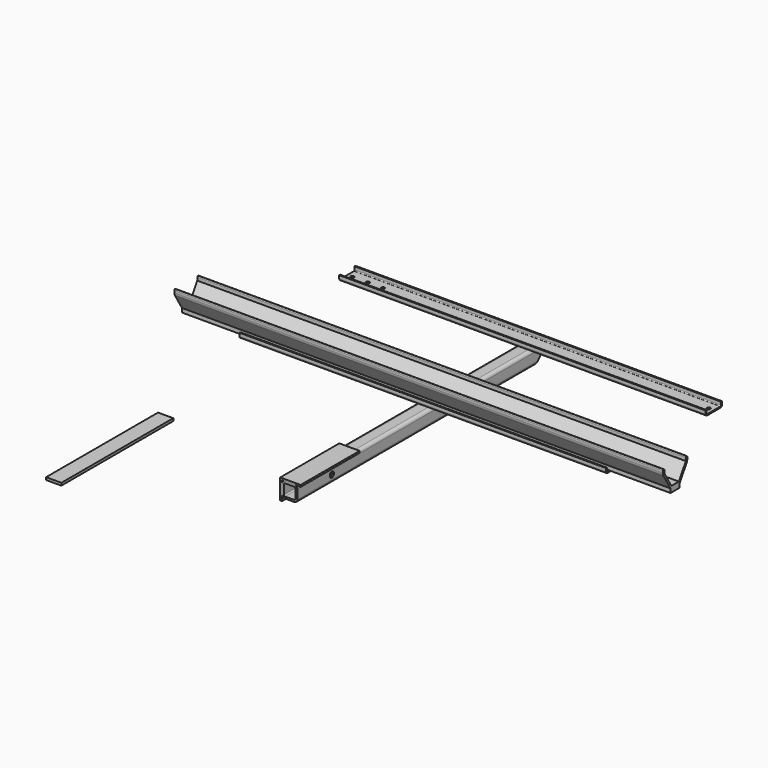
from build123d import *

# Parameters (mm, degrees)
F0_W         = 38.1
F0_H         = 38.1
F1_DEPTH     = 781.05
F2_R         = 7.62
F3_T         = -4.6228
F5_DEPTH     = 19.05
F7_DEPTH     = 184.15
F9_D         = 13.49248
F9_2_D       = 13.49248
F10_W        = 50.8
F10_H        = 12.7
F11_DEPTH    = 457.2
F12_R        = 5.08
F13_T        = -2.9972
F15_D        = 8.4328
F17_ANGLE    = 180
F18_W        = 38.1
F18_H        = 349.25
F19_DEPTH    = 6.35
F21_DEPTH    = 609.6
F22_T        = -4.572
F20_W        = 28.575
F20_H        = 10.1452730596
F23_DEPTH    = 609.6
F24_T1_DEPTH = 1231.9
F25_R        = 12.7
F27_DEPTH    = 7.62


# Not quite as in the source:
# - a fillet or chamfer that OpenCascade refuses, or shapes differently, is made with other operations: its cross-section is extruded or revolved along the edge and cut away or added


with BuildPart() as f1:
    # F0 (on Front) → F1 (new body)
    with BuildSketch(Plane.XZ):
        Rectangle(F0_W, F0_H)
    extrude(amount=-F1_DEPTH)

    # F2
    f2_edges = [f1.edges().sort_by_distance(p)[0] for p in [
        (-19.05, 390.525, -19.05),
        (-19.05, 390.525, 19.05),
        (19.05, 390.525, -19.05),
        (19.05, 390.525, 19.05),
    ]]
    fillet(f2_edges, radius=F2_R)

    # F3
    f3_openings = [f1.faces().sort_by_distance(p)[0] for p in [
        (0, 781.05, 0),
        (0, 0, 0),
    ]]
    offset(amount=F3_T, openings=f3_openings)

    # F4 (on Right) → F5 (cut, symmetric)
    with BuildSketch(Plane.YZ):
        Polygon((781.05, -19.05), (781.05, -14.4272), (781.05, 14.4272), (781.05, 19.05), (742.95, -19.05), align=None)
    extrude(amount=F5_DEPTH, both=True, mode=Mode.SUBTRACT)

    # F9 (through all)
    with Locations(Plane.YZ.offset(19.05)):
        with Locations((107.95, 0)):
            Hole(F9_D / 2)


with BuildPart() as f7:
    # F6 (on Front) → F7 (new body)
    with BuildSketch(Plane.XZ):
        Polygon((27.178, 23.622), (-23.622, 23.622), (-23.622, -27.178), (-19.05, -27.178), (-19.05, 19.05), (27.178, 19.05), align=None)
    extrude(amount=-F7_DEPTH)

    # F9#2 (through all)
    with Locations(Plane.YZ.offset(19.05)):
        with Locations((107.95, 0)):
            Hole(F9_2_D / 2)


with BuildPart() as f11:
    # F10 (on Right) → F11 (new body, symmetric)
    with BuildSketch(Plane.YZ):
        with Locations((751.332, 25.4)):
            Rectangle(F10_W, F10_H)
    extrude(amount=F11_DEPTH, both=True)

    # F12
    f12_edges = [f11.edges().sort_by_distance(p)[0] for p in [
        (0, 725.932, 19.05),
        (0, 776.732, 19.05),
    ]]
    fillet(f12_edges, radius=F12_R)

    # F13
    f13_openings = [f11.faces().sort_by_distance(p)[0] for p in [
        (0, 751.332, 31.75),
        (457.2, 751.332, 25.491101),
        (-457.2, 751.332, 25.491101),
    ]]
    offset(amount=F13_T, openings=f13_openings)

    # F15 (through all)
    with Locations(Plane.XY.offset(22.0472)):
        with Locations((406.4, 751.332), (368.3, 751.332), (444.5, 751.332), (-444.5, 751.332)):
            Hole(F15_D / 2)


with BuildPart() as f16_1:
    # F16: copy of F11
    add(f11.part.moved(Location((0, -311.15, 0))))


with BuildPart() as f11_1:
    # F17: moved
    add(f11.part.rotate(Axis((0, 751.332, 25.4), (0, 0, 1)), F17_ANGLE))


with BuildPart() as f19:
    # F18 (on face) → F19 (new body)
    with BuildSketch(Plane(origin=(0, 0, 19.05), x_dir=(1, 0, 0), z_dir=(0, 0, -1))):
        with Locations((-367.03, 102.743)):
            Rectangle(F18_W, F18_H)
    extrude(amount=F19_DEPTH)


with BuildPart() as f21:
    # F20 (on Right) → F21 (new body, symmetric)
    with BuildSketch(Plane.YZ):
        Polygon((402.082, 71.5478807688), (425.8945, 32.1924730596), (454.4695, 32.1924730596), (478.282, 71.5478807688), (478.282, 82.9924730596), (402.082, 82.9924730596), align=None)
    extrude(amount=F21_DEPTH, both=True)

    # F22
    f22_openings = [f21.faces().sort_by_distance(p)[0] for p in [
        (609.6, 440.182, 61.515579),
        (0, 440.182, 82.992473),
        (-609.6, 440.182, 61.515579),
    ]]
    offset(amount=F22_T, openings=f22_openings)

    # F20 (on Right) → F23 (join, symmetric)
    with BuildSketch(Plane.YZ):
        with Locations((440.182, 27.1198365298)):
            Rectangle(F20_W, F20_H)
    extrude(amount=F23_DEPTH, both=True)

    # F24: fillet of radius 2.54 on 4 edges, made by hand

    # F24_s2 → F24_t1 (cut)
    with BuildSketch(Plane.YZ.offset(-615.95)):
        with BuildLine():
            ThreePointArc((478.282, 80.4524730596), (477.5380512242, 82.2485242838), (475.742, 82.9924730596))
            Line((475.742, 82.9924730596), (478.282, 82.9924730596))
            Line((478.282, 82.9924730596), (478.282, 80.4524730596))
        make_face()
        with BuildLine():
            ThreePointArc((476.25, 82.9924730596), (474.4539487758, 82.2485242838), (473.71, 80.4524730596))
            Line((473.71, 80.4524730596), (473.71, 82.9924730596))
            Line((473.71, 82.9924730596), (476.25, 82.9924730596))
        make_face()
        with BuildLine():
            ThreePointArc((402.082, 80.4524730596), (402.8259487758, 82.2485242838), (404.622, 82.9924730596))
            Line((404.622, 82.9924730596), (402.082, 82.9924730596))
            Line((402.082, 82.9924730596), (402.082, 80.4524730596))
        make_face()
        with BuildLine():
            ThreePointArc((406.654, 80.4524730596), (405.9100512242, 82.2485242838), (404.114, 82.9924730596))
            Line((404.114, 82.9924730596), (406.654, 82.9924730596))
            Line((406.654, 82.9924730596), (406.654, 80.4524730596))
        make_face()
    extrude(amount=F24_T1_DEPTH, mode=Mode.SUBTRACT)

    # F25
    f25_edges = [f21.edges().sort_by_distance(p)[0] for p in [
        (0, 478.282, 71.547881),
        (0, 402.082, 71.547881),
    ]]
    fillet(f25_edges, radius=F25_R)

    # F26 (on face) → F27 (cut)
    with BuildSketch(Plane(origin=(0, 0, 22.0472), x_dir=(1, 0, 0), z_dir=(0, 0, -1))):
        with BuildLine():
            ThreePointArc((596.9, -444.119), (600.837, -440.182), (596.9, -436.245))
            Line((596.9, -436.245), (-596.9, -436.245))
            ThreePointArc((-596.9, -436.245), (-600.837, -440.182), (-596.9, -444.119))
            Line((-596.9, -444.119), (596.9, -444.119))
        make_face()
    extrude(amount=-F27_DEPTH, mode=Mode.SUBTRACT)


solid = Compound([f1.part, f7.part, f16_1.part, f11_1.part, f19.part, f21.part])
